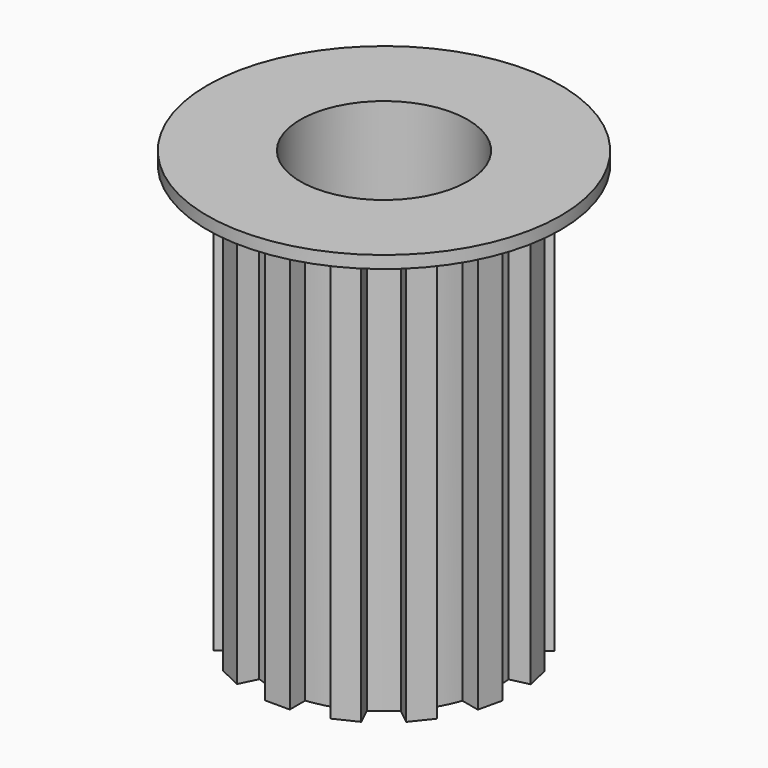
from build123d import *

# Parameters (mm, degrees)
F0_R            = 9.25
F0_R_2          = 6.75
F1_DEPTH        = 35
F2_W            = 2
F2_H            = 3
F3_DEPTH        = 35
F3_COPIES_COUNT = 14
F4_R            = 14.25
F4_R_2          = 6.75
F5_DEPTH        = 1


# Not quite as in the source:
# - a pattern or mirror of a feature is missing from the dataset's text; its kind, count and spacing are read off the source's solid


with BuildPart() as f1:
    # F0 (on Top) → F1 (new body)
    with BuildSketch(Plane.XY):
        Circle(F0_R)
        Circle(F0_R_2, mode=Mode.SUBTRACT)
    extrude(amount=F1_DEPTH)

    # F2 (on face) → F3 (join)
    with BuildSketch(Plane.XY.offset(35)):
        with Locations((0, 9.25)):
            Rectangle(F2_W, F2_H)
    f3 = extrude(amount=-F3_DEPTH)

    # F3_copies: F3 ×14 about axis
    f3_copies_axis = Axis((0, 0, 0), (0, 0, 1))
    for i in range(1, F3_COPIES_COUNT):
        add(f3.rotate(f3_copies_axis, i * 360 / F3_COPIES_COUNT))

    # F4 (on face) → F5 (join)
    with BuildSketch(Plane.XY.offset(35)):
        Circle(F4_R)
        Circle(F4_R_2, mode=Mode.SUBTRACT)
    extrude(amount=-F5_DEPTH)


solid = f1.part
